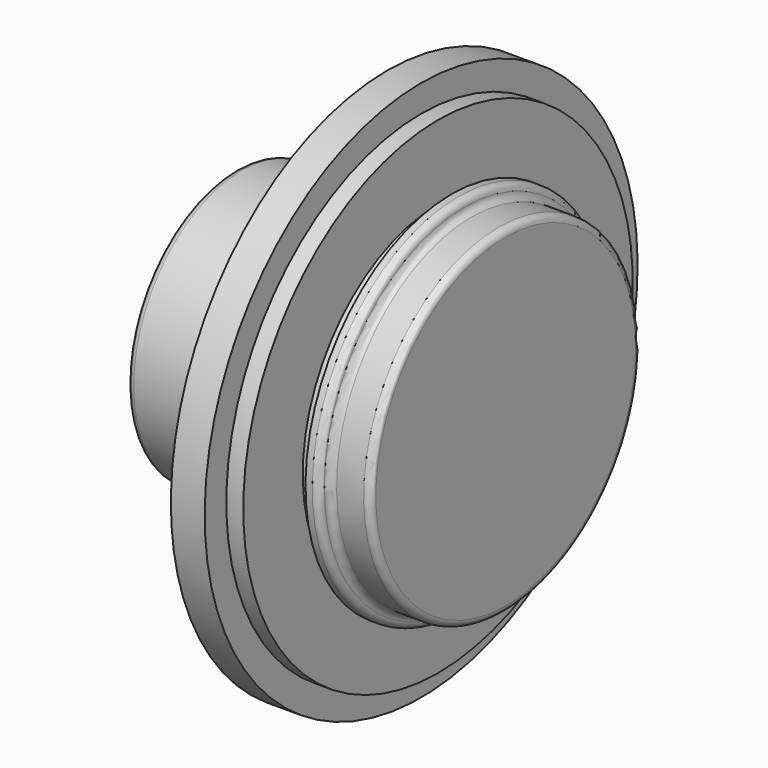
from build123d import *

# Parameters (mm, degrees)
F2_R = 0.49999


# Not quite as in the source:
# - a fillet or chamfer is up to 0.001 mm smaller than in the source, because OpenCascade refuses the exact size


with BuildPart() as f1:
    # F0 (on Front) → F1 (revolve)
    with BuildSketch(Plane.XZ):
        Polygon((-20, 0), (0, 0), (0, 12.5), (-3, 12.5), (-3, 13.5), (-4, 13.5), (-4, 12.5), (-5, 12.5), (-5, 18), (-6.25, 18), (-6.25, 20), (-8.75, 20), (-8.75, 18), (-10, 18), (-10, 10), (-20, 10), align=None)
    revolve(axis=Axis((-10, 0, 0), (-1, 0, 0)))

    # F2 (radius 0.5 in the source; OpenCascade refuses exactly that, so slightly less here)
    f2_edges = [f1.edges().sort_by_distance(p)[0] for p in [
        (-20, 0, -10),
        (-3, 0, -13.5),
        (0, 0, -12.5),
        (-3, 0, -12.5),
        (-1.5, 0, 12.5),
    ]]
    fillet(f2_edges, radius=F2_R)


solid = f1.part
